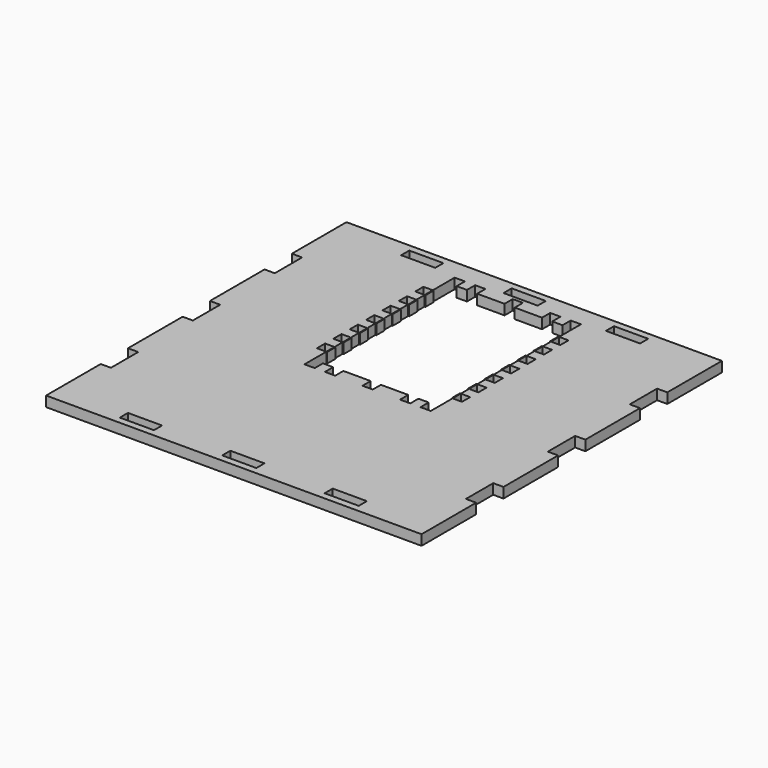
from build123d import *

# Parameters (mm, degrees)
F0_W     = 10
F0_H     = 2.98
F1_DEPTH = 3
F2_W     = 3
F2_H     = 3
F2_W_2   = 2.75
F2_W_3   = 19.4
F2_H_2   = 39.9
F3_DEPTH = 25


with BuildPart() as f1:
    # F0 (on Top) → F1 (new body)
    with BuildSketch(Plane.XY):
        Polygon((52, 34.99), (55, 34.99), (55, 54.99), (-55, 54.99), (-55, 34.99), (-52, 34.99), (-52, 24.99), (-55, 24.99), (-55, 4.99), (-52, 4.99), (-52, -5.01), (-55, -5.01), (-55, -25.01), (-52, -25.01), (-52, -35.01), (-55, -35.01), (-55, -55.01), (55, -55.01), (55, -35.01), (52, -35.01), (52, -25.01), (55, -25.01), (55, -5.01), (52, -5.01), (52, 4.99), (55, 4.99), (55, 24.99), (52, 24.99), align=None)
        with Locations((-30, -51.52)):
            Rectangle(F0_W, F0_H, mode=Mode.SUBTRACT)
        with Locations((0, -51.52)):
            Rectangle(F0_W, F0_H, mode=Mode.SUBTRACT)
        with Locations((30, -51.52)):
            Rectangle(F0_W, F0_H, mode=Mode.SUBTRACT)
        with Locations((-30, 51.5)):
            Rectangle(F0_W, F0_H, mode=Mode.SUBTRACT)
        with Locations((0, 51.5)):
            Rectangle(F0_W, F0_H, mode=Mode.SUBTRACT)
        with Locations((30, 51.5)):
            Rectangle(F0_W, F0_H, mode=Mode.SUBTRACT)
    extrude(amount=F1_DEPTH)

    # F2 (on face) → F3 (cut)
    with BuildSketch(Plane.XY.offset(3)):
        with Locations((17, -4.51)):
            Rectangle(F2_W, F2_H)
        with Locations((19.875, 3.49)):
            Rectangle(F2_W_2, F2_H)
        with BuildLine():
            Line((15.5, -3.01), (18.5, -3.01))
            Line((18.5, -3.01), (18.5, 1.99))
            Line((18.5, 1.99), (18.25, 1.99))
            Line((18.25, 1.99), (18.25, 4.99))
            Line((18.25, 4.99), (18.5, 4.99))
            Line((18.5, 4.99), (18.5, 7.99))
            Line((18.5, 7.99), (18.25, 7.99))
            Line((18.25, 7.99), (18.25, 10.99))
            Line((18.25, 10.99), (18.5, 10.99))
            Line((18.5, 10.99), (18.5, 13.99))
            Line((18.5, 13.99), (18.25, 13.99))
            Line((18.25, 13.99), (18.25, 16.99))
            Line((18.25, 16.99), (18.5, 16.99))
            Line((18.5, 16.99), (18.5, 19.99))
            Line((18.5, 19.99), (18.25, 19.99))
            Line((18.25, 19.99), (18.25, 22.99))
            Line((18.25, 22.99), (18.5, 22.99))
            Line((18.5, 22.99), (18.5, 25.99))
            Line((18.5, 25.99), (18.25, 25.99))
            Line((18.25, 25.99), (18.25, 28.99))
            Line((18.25, 28.99), (18.5, 28.99))
            Line((18.5, 28.99), (18.5, 31.99))
            Line((18.5, 31.99), (18.25, 31.99))
            Line((18.25, 31.99), (18.25, 34.99))
            Line((18.25, 34.99), (18.5, 34.99))
            Line((18.5, 34.99), (18.5, 37.99))
            Line((18.5, 37.99), (18.25, 37.99))
            Line((18.25, 37.99), (18.25, 40.99))
            Line((18.25, 40.99), (18.5, 40.99))
            Line((18.5, 40.99), (18.5, 45.99))
            Line((18.5, 45.99), (15.5, 45.99))
            Line((15.5, 45.99), (12.5, 45.99))
            Line((12.5, 45.99), (9.5, 45.99))
            Line((9.5, 45.99), (6.5724185194, 45.99))
            ThreePointArc((6.5724185194, 45.99), (6.6304892758, 45.7429915444), (6.65, 45.49))
            ThreePointArc((6.65, 45.49), (4.7470084556, 43.8595107242), (3.4275814806, 45.99))
            Line((3.4275814806, 45.99), (1.5, 45.99))
            Line((1.5, 45.99), (-1.5, 45.99))
            Line((-1.5, 45.99), (-3.4275814806, 45.99))
            ThreePointArc((-3.4275814806, 45.99), (-3.3695107242, 45.7429915444), (-3.35, 45.49))
            ThreePointArc((-3.35, 45.49), (-5.2529915444, 43.8595107242), (-6.5724185194, 45.99))
            Line((-6.5724185194, 45.99), (-9.5, 45.99))
            Line((-9.5, 45.99), (-12.5, 45.99))
            Line((-12.5, 45.99), (-15.5, 45.99))
            Line((-15.5, 45.99), (-18.5, 45.99))
            Line((-18.5, 45.99), (-18.5, 40.99))
            Line((-18.5, 40.99), (-18.25, 40.99))
            Line((-18.25, 40.99), (-18.25, 37.99))
            Line((-18.25, 37.99), (-18.5, 37.99))
            Line((-18.5, 37.99), (-18.5, 34.99))
            Line((-18.5, 34.99), (-18.25, 34.99))
            Line((-18.25, 34.99), (-18.25, 31.99))
            Line((-18.25, 31.99), (-18.5, 31.99))
            Line((-18.5, 31.99), (-18.5, 28.99))
            Line((-18.5, 28.99), (-18.25, 28.99))
            Line((-18.25, 28.99), (-18.25, 25.99))
            Line((-18.25, 25.99), (-18.5, 25.99))
            Line((-18.5, 25.99), (-18.5, 22.99))
            Line((-18.5, 22.99), (-18.25, 22.99))
            Line((-18.25, 22.99), (-18.25, 19.99))
            Line((-18.25, 19.99), (-18.5, 19.99))
            Line((-18.5, 19.99), (-18.5, 16.99))
            Line((-18.5, 16.99), (-18.25, 16.99))
            Line((-18.25, 16.99), (-18.25, 13.99))
            Line((-18.25, 13.99), (-18.5, 13.99))
            Line((-18.5, 13.99), (-18.5, 10.99))
            Line((-18.5, 10.99), (-18.25, 10.99))
            Line((-18.25, 10.99), (-18.25, 7.99))
            Line((-18.25, 7.99), (-18.5, 7.99))
            Line((-18.5, 7.99), (-18.5, 4.99))
            Line((-18.5, 4.99), (-18.25, 4.99))
            Line((-18.25, 4.99), (-18.25, 1.99))
            Line((-18.25, 1.99), (-18.5, 1.99))
            Line((-18.5, 1.99), (-18.5, -3.01))
            Line((-18.5, -3.01), (-15.5, -3.01))
            Line((-15.5, -3.01), (-12.5, -3.01))
            Line((-12.5, -3.01), (-9.5, -3.01))
            Line((-9.5, -3.01), (-6.5724185194, -3.01))
            ThreePointArc((-6.5724185194, -3.01), (-5.2529915444, -0.8795107242), (-3.35, -2.51))
            ThreePointArc((-3.35, -2.51), (-3.3695107242, -2.7629915444), (-3.4275814806, -3.01))
            Line((-3.4275814806, -3.01), (-1.5, -3.01))
            Line((-1.5, -3.01), (1.5, -3.01))
            Line((1.5, -3.01), (3.4275814806, -3.01))
            ThreePointArc((3.4275814806, -3.01), (4.7470084556, -0.8795107242), (6.65, -2.51))
            ThreePointArc((6.65, -2.51), (6.6304892758, -2.7629915444), (6.5724185194, -3.01))
            Line((6.5724185194, -3.01), (9.5, -3.01))
            Line((9.5, -3.01), (12.5, -3.01))
            Line((12.5, -3.01), (15.5, -3.01))
        make_face()
        with Locations((0, 21.49)):
            Rectangle(F2_W_3, F2_H_2, mode=Mode.SUBTRACT)
        with Locations((11, -4.51)):
            Rectangle(F2_W, F2_H)
        with Locations((19.875, 9.49)):
            Rectangle(F2_W_2, F2_H)
        with Locations((0, -4.51)):
            Rectangle(F2_W, F2_H)
        with Locations((19.875, 15.49)):
            Rectangle(F2_W_2, F2_H)
        with BuildLine():
            Line((3.4275814806, -3.01), (6.5724185194, -3.01))
            ThreePointArc((6.5724185194, -3.01), (6.6304892758, -2.7629915444), (6.65, -2.51))
            ThreePointArc((6.65, -2.51), (4.7470084556, -0.8795107242), (3.4275814806, -3.01))
        make_face()
        with Locations((-11, -4.51)):
            Rectangle(F2_W, F2_H)
        with Locations((19.875, 21.49)):
            Rectangle(F2_W_2, F2_H)
        with BuildLine():
            Line((-6.5724185194, -3.01), (-3.4275814806, -3.01))
            ThreePointArc((-3.4275814806, -3.01), (-3.3695107242, -2.7629915444), (-3.35, -2.51))
            ThreePointArc((-3.35, -2.51), (-5.2529915444, -0.8795107242), (-6.5724185194, -3.01))
        make_face()
        with Locations((-17, -4.51)):
            Rectangle(F2_W, F2_H)
        with Locations((19.875, 27.49)):
            Rectangle(F2_W_2, F2_H)
        with Locations((19.875, 33.49)):
            Rectangle(F2_W_2, F2_H)
        with Locations((-19.875, 3.49)):
            Rectangle(F2_W_2, F2_H)
        with Locations((19.875, 39.49)):
            Rectangle(F2_W_2, F2_H)
        with Locations((-19.875, 9.49)):
            Rectangle(F2_W_2, F2_H)
        with Locations((-19.875, 15.49)):
            Rectangle(F2_W_2, F2_H)
        with Locations((17, 47.49)):
            Rectangle(F2_W, F2_H)
        with Locations((-19.875, 21.49)):
            Rectangle(F2_W_2, F2_H)
        with Locations((11, 47.49)):
            Rectangle(F2_W, F2_H)
        with Locations((-19.875, 27.49)):
            Rectangle(F2_W_2, F2_H)
        with Locations((0, 47.49)):
            Rectangle(F2_W, F2_H)
        with BuildLine():
            ThreePointArc((6.65, 45.49), (6.6304892758, 45.7429915444), (6.5724185194, 45.99))
            Line((6.5724185194, 45.99), (3.4275814806, 45.99))
            ThreePointArc((3.4275814806, 45.99), (4.7470084556, 43.8595107242), (6.65, 45.49))
        make_face()
        with Locations((-19.875, 33.49)):
            Rectangle(F2_W_2, F2_H)
        with Locations((-11, 47.49)):
            Rectangle(F2_W, F2_H)
        with BuildLine():
            ThreePointArc((-3.35, 45.49), (-3.3695107242, 45.7429915444), (-3.4275814806, 45.99))
            Line((-3.4275814806, 45.99), (-6.5724185194, 45.99))
            ThreePointArc((-6.5724185194, 45.99), (-5.2529915444, 43.8595107242), (-3.35, 45.49))
        make_face()
        with Locations((-19.875, 39.49)):
            Rectangle(F2_W_2, F2_H)
        with Locations((-17, 47.49)):
            Rectangle(F2_W, F2_H)
        with Locations((0, 21.49)):
            Rectangle(F2_W_3, F2_H_2)
    extrude(amount=-F3_DEPTH, mode=Mode.SUBTRACT)


solid = f1.part
